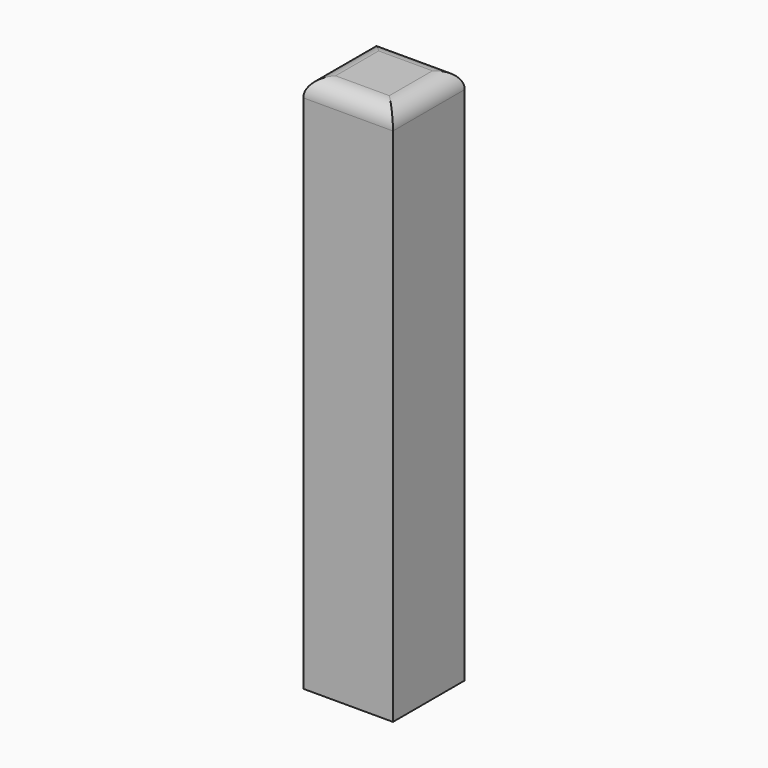
from build123d import *

# Parameters (mm, degrees)
F0_W     = 10
F0_H     = 60
F1_DEPTH = 10
F3_D     = 4.4
F3_DEPTH = 3.6
F3_TIP   = 1.3218933619
F4_R     = 2


with BuildPart() as f1:
    # F0 (on Front) → F1 (new body)
    with BuildSketch(Plane.XZ):
        Rectangle(F0_W, F0_H)
    extrude(amount=F1_DEPTH)

    # F3
    with Locations(Plane(origin=(0, 0, -30), x_dir=(1, 0, 0), z_dir=(0, 0, -1))):
        with Locations((0, 5.1514371298)):
            Hole(F3_D / 2, depth=F3_DEPTH)
            with Locations((0, 0, -(F3_DEPTH + F3_TIP / 2))):  # 118° drill point
                Cone(0, F3_D / 2, F3_TIP, mode=Mode.SUBTRACT)

    # F4
    f4_edges = [f1.edges().sort_by_distance(p)[0] for p in [
        (5, -5, 30),
        (-5, -5, 30),
        (0, 0, 30),
        (0, -10, 30),
    ]]
    fillet(f4_edges, radius=F4_R)


solid = f1.part
